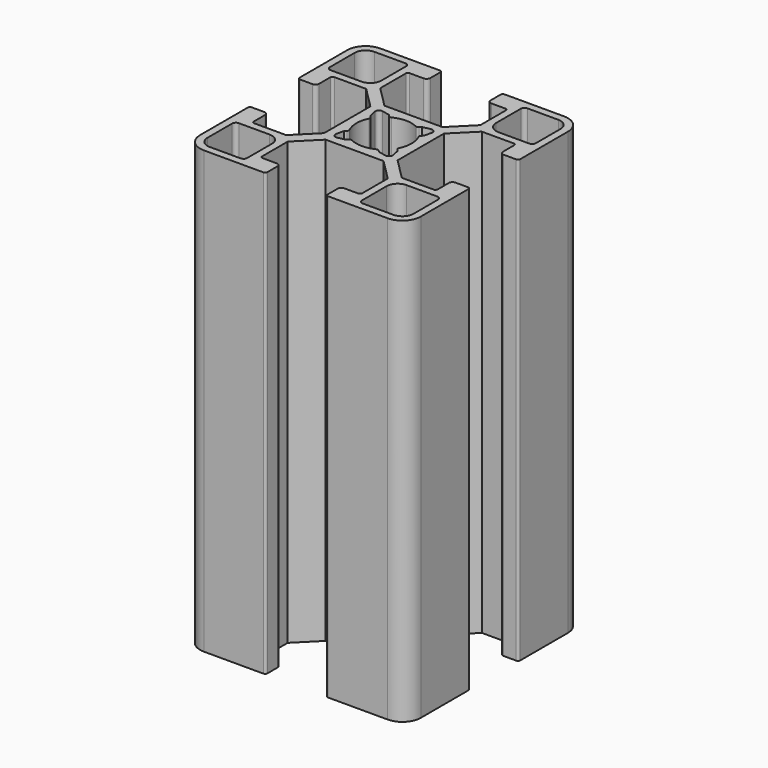
from build123d import *

# Parameters (mm, degrees)
F1_DEPTH = 60


# Not quite as in the source:
# - ends of sketch curves that miss each other by under 0.0002 mm in the source are joined
# - the program builds the solid bodies; features that only make, move or delete a surface that nothing else refers to are left out


with BuildPart() as f1:
    # F0 (on Top) → F1 (new body)
    with BuildSketch(Plane.XY):
        with BuildLine():
            Line((3.939341, -5), (6.799995, -7.860656))
            Line((6.799995, -7.860656), (6.799995, -12.199997))
            ThreePointArc((6.799995, -12.199997), (6.7121307415, -12.4121300846), (6.5, -12.5))
            Line((6.5, -12.5), (4.599998, -12.5))
            ThreePointArc((4.599998, -12.5), (4.2464446094, -12.6464466094), (4.099998, -13))
            Line((4.099998, -13), (4.099998, -14.699997))
            ThreePointArc((4.099998, -14.699997), (4.1878632585, -14.9121300846), (4.399994, -15))
            Line((4.399994, -15), (12.5, -15))
            ThreePointArc((12.5, -15), (14.267766953, -14.267766953), (15, -12.5))
            Line((15, -12.5), (15, -4.399994))
            ThreePointArc((15, -4.399994), (14.9121300846, -4.1878632585), (14.699997, -4.099999))
            Line((14.699997, -4.099999), (13, -4.099998))
            ThreePointArc((13, -4.099998), (12.6464466094, -4.2464446094), (12.5, -4.599998))
            Line((12.5, -4.599998), (12.5, -6.5))
            ThreePointArc((12.5, -6.5), (12.4121300846, -6.7121307415), (12.199997, -6.799995))
            Line((12.199997, -6.799995), (7.860655, -6.799995))
            Line((7.860655, -6.799995), (5, -3.93934))
            Line((5, -3.93934), (5, 3.939341))
            Line((5, 3.939341), (7.860655, 6.799995))
            Line((7.860655, 6.799995), (12.199997, 6.799995))
            ThreePointArc((12.199997, 6.799995), (12.4121300846, 6.7121307415), (12.5, 6.5))
            Line((12.5, 6.5), (12.5, 4.599998))
            ThreePointArc((12.5, 4.599998), (12.6464466094, 4.2464446094), (13, 4.099998))
            Line((13, 4.099998), (14.699997, 4.099998))
            ThreePointArc((14.699997, 4.099998), (14.9121300846, 4.1878632585), (15, 4.399994))
            Line((15, 4.399994), (15, 12.5))
            ThreePointArc((15, 12.5), (14.267766953, 14.267766953), (12.5, 15))
            Line((12.5, 15), (4.399994, 15))
            ThreePointArc((4.399994, 15), (4.1878632585, 14.9121300846), (4.099999, 14.699997))
            Line((4.099999, 14.699997), (4.099998, 13))
            ThreePointArc((4.099998, 13), (4.2464446094, 12.6464466094), (4.599998, 12.5))
            Line((4.599998, 12.5), (6.5, 12.5))
            ThreePointArc((6.5, 12.5), (6.7121307415, 12.4121300846), (6.799995, 12.199997))
            Line((6.799995, 12.199997), (6.799995, 7.860655))
            Line((6.799995, 7.860655), (3.939341, 5))
            Line((3.939341, 5), (-3.93934, 5))
            Line((-3.93934, 5), (-6.799995, 7.860655))
            Line((-6.799995, 7.860655), (-6.799995, 12.199997))
            ThreePointArc((-6.799995, 12.199997), (-6.7121307415, 12.4121300846), (-6.5, 12.5))
            Line((-6.5, 12.5), (-4.599998, 12.5))
            ThreePointArc((-4.599998, 12.5), (-4.2464446094, 12.6464466094), (-4.099998, 13))
            Line((-4.099998, 13), (-4.099998, 14.699997))
            ThreePointArc((-4.099998, 14.699997), (-4.1878632585, 14.9121300846), (-4.399994, 15))
            Line((-4.399994, 15), (-12.5, 15))
            ThreePointArc((-12.5, 15), (-14.267766953, 14.267766953), (-15, 12.5))
            Line((-15, 12.5), (-15, 4.399994))
            ThreePointArc((-15, 4.399994), (-14.9121300846, 4.1878632585), (-14.699997, 4.099999))
            Line((-14.699997, 4.099999), (-13, 4.099998))
            ThreePointArc((-13, 4.099998), (-12.6464466094, 4.2464446094), (-12.5, 4.599998))
            Line((-12.5, 4.599998), (-12.5, 6.5))
            ThreePointArc((-12.5, 6.5), (-12.4121300846, 6.7121307415), (-12.199997, 6.799995))
            Line((-12.199997, 6.799995), (-7.860656, 6.799995))
            Line((-7.860656, 6.799995), (-5, 3.939341))
            Line((-5, 3.939341), (-5, -3.93934))
            Line((-5, -3.93934), (-7.860656, -6.799995))
            Line((-7.860656, -6.799995), (-12.199997, -6.799995))
            ThreePointArc((-12.199997, -6.799995), (-12.4121300846, -6.7121307415), (-12.5, -6.5))
            Line((-12.5, -6.5), (-12.5, -4.599998))
            ThreePointArc((-12.5, -4.599998), (-12.6464466094, -4.2464446094), (-13, -4.099998))
            Line((-13, -4.099998), (-14.699997, -4.099998))
            ThreePointArc((-14.699997, -4.099998), (-14.9121300846, -4.1878632585), (-15, -4.399994))
            Line((-15, -4.399994), (-15, -12.5))
            ThreePointArc((-15, -12.5), (-14.267766953, -14.267766953), (-12.5, -15))
            Line((-12.5, -15), (-4.399994, -15))
            ThreePointArc((-4.399994, -15), (-4.1878632585, -14.9121300846), (-4.099999, -14.699997))
            Line((-4.099999, -14.699997), (-4.099998, -13))
            ThreePointArc((-4.099998, -13), (-4.2464446094, -12.6464466094), (-4.599998, -12.5))
            Line((-4.599998, -12.5), (-6.5, -12.5))
            ThreePointArc((-6.5, -12.5), (-6.7121307415, -12.4121300846), (-6.799995, -12.199997))
            Line((-6.799995, -12.199997), (-6.799995, -7.860656))
            Line((-6.799995, -7.860656), (-3.93934, -5))
            Line((-3.93934, -5), (3.939341, -5))
        make_face()
        with BuildLine():
            Line((-8.299995, -14), (-12.5, -14))
            ThreePointArc((-12.5, -14), (-13.5606601718, -13.5606601718), (-14, -12.5))
            Line((-14, -12.5), (-14, -8.299995))
            ThreePointArc((-14, -8.299995), (-13.8535533906, -7.9464416094), (-13.5, -7.799995))
            Line((-13.5, -7.799995), (-9.299995, -7.799995))
            ThreePointArc((-9.299995, -7.799995), (-8.2393348282, -8.2393348282), (-7.799995, -9.299995))
            Line((-7.799995, -9.299995), (-7.799995, -13.5))
            ThreePointArc((-7.799995, -13.5), (-7.9464416094, -13.8535533906), (-8.299995, -14))
        make_face(mode=Mode.SUBTRACT)
        with BuildLine():
            Line((12.5, -14), (8.299995, -14))
            ThreePointArc((8.299995, -14), (7.9464416094, -13.8535533906), (7.799995, -13.5))
            Line((7.799995, -13.5), (7.799995, -9.299995))
            ThreePointArc((7.799995, -9.299995), (8.2393348282, -8.2393348282), (9.299995, -7.799995))
            Line((9.299995, -7.799995), (13.5, -7.799995))
            ThreePointArc((13.5, -7.799995), (13.8535533906, -7.9464416094), (14, -8.299995))
            Line((14, -8.299995), (14, -12.5))
            ThreePointArc((14, -12.5), (13.5606601718, -13.5606601718), (12.5, -14))
        make_face(mode=Mode.SUBTRACT)
        with BuildLine():
            Line((3.657288, -2.243073), (3.878887, -3.285876))
            ThreePointArc((3.878887, -3.285876), (3.7433613906, -3.7433613906), (3.2858769836, -3.8788870773))
            Line((3.2858769836, -3.8788870773), (2.243074, -3.657287))
            Line((2.243074, -3.657287), (2.005135, -3.419348))
            ThreePointArc((2.005135, -3.419348), (1.841799908, -3.3354753308), (1.6601868142, -3.3624816237))
            ThreePointArc((1.6601868142, -3.3624816237), (0, -3.75), (-1.6601870383, -3.3624810777))
            ThreePointArc((-1.6601870383, -3.3624810777), (-1.841799908, -3.3354753308), (-2.0051340344, -3.4193479656))
            Line((-2.0051340344, -3.4193479656), (-2.243073, -3.657287))
            Line((-2.243073, -3.657287), (-3.285876, -3.878887))
            ThreePointArc((-3.285876, -3.878887), (-3.7433613906, -3.7433613906), (-3.8788870773, -3.2858769836))
            Line((-3.8788870773, -3.2858769836), (-3.657287, -2.243073))
            Line((-3.657287, -2.243073), (-3.419348, -2.005134))
            ThreePointArc((-3.419348, -2.005134), (-3.3354753308, -1.841799908), (-3.3624816237, -1.6601868142))
            ThreePointArc((-3.3624816237, -1.6601868142), (-3.75, 0), (-3.3624810777, 1.6601870383))
            ThreePointArc((-3.3624810777, 1.6601870383), (-3.3354753883, 1.8418002569), (-3.4193484656, 2.0051345344))
            Line((-3.4193484656, 2.0051345344), (-3.657287, 2.243074))
            Line((-3.657287, 2.243074), (-3.878887, 3.285877))
            ThreePointArc((-3.878887, 3.285877), (-3.7433613906, 3.7433613906), (-3.2858769836, 3.8788870773))
            Line((-3.2858769836, 3.8788870773), (-2.243073, 3.657288))
            Line((-2.243073, 3.657288), (-2.005134, 3.419348))
            ThreePointArc((-2.005134, 3.419348), (-1.8418001264, 3.3354753668), (-1.6601872112, 3.3624814277))
            ThreePointArc((-1.6601872112, 3.3624814277), (0, 3.75), (1.6601870383, 3.3624810777))
            ThreePointArc((1.6601870383, 3.3624810777), (1.8418002569, 3.3354753883), (2.0051345344, 3.4193484656))
            Line((2.0051345344, 3.4193484656), (2.243074, 3.657288))
            Line((2.243074, 3.657288), (3.285877, 3.878887))
            ThreePointArc((3.285877, 3.878887), (3.7433610448, 3.7433617364), (3.8788872806, 3.2858779404))
            Line((3.8788872806, 3.2858779404), (3.657288, 2.243074))
            Line((3.657288, 2.243074), (3.419348, 2.005135))
            ThreePointArc((3.419348, 2.005135), (3.3354753668, 1.8418001264), (3.3624814277, 1.6601872112))
            ThreePointArc((3.3624814277, 1.6601872112), (3.75, 0), (3.3624810777, -1.6601870383))
            ThreePointArc((3.3624810777, -1.6601870383), (3.3354753308, -1.841799908), (3.4193479656, -2.0051340344))
            Line((3.4193479656, -2.0051340344), (3.657288, -2.243073))
        make_face(mode=Mode.SUBTRACT)
        with BuildLine():
            Line((-9.299995, 7.799995), (-13.5, 7.799995))
            ThreePointArc((-13.5, 7.799995), (-13.8535533906, 7.9464416094), (-14, 8.299995))
            Line((-14, 8.299995), (-14, 12.5))
            ThreePointArc((-14, 12.5), (-13.5606601718, 13.5606601718), (-12.5, 14))
            Line((-12.5, 14), (-8.299995, 14))
            ThreePointArc((-8.299995, 14), (-7.9464416094, 13.8535533906), (-7.799995, 13.5))
            Line((-7.799995, 13.5), (-7.799995, 9.299995))
            ThreePointArc((-7.799995, 9.299995), (-8.2393348282, 8.2393348282), (-9.299995, 7.799995))
        make_face(mode=Mode.SUBTRACT)
        with BuildLine():
            Line((13.5, 7.799995), (9.299995, 7.799995))
            ThreePointArc((9.299995, 7.799995), (8.2393348282, 8.2393348282), (7.799995, 9.299995))
            Line((7.799995, 9.299995), (7.799995, 13.5))
            ThreePointArc((7.799995, 13.5), (7.9464416094, 13.8535533906), (8.299995, 14))
            Line((8.299995, 14), (12.5, 14))
            ThreePointArc((12.5, 14), (13.5606601718, 13.5606601718), (14, 12.5))
            Line((14, 12.5), (14, 8.299995))
            ThreePointArc((14, 8.299995), (13.8535533906, 7.9464416094), (13.5, 7.799995))
        make_face(mode=Mode.SUBTRACT)
    extrude(amount=F1_DEPTH)


solid = f1.part
